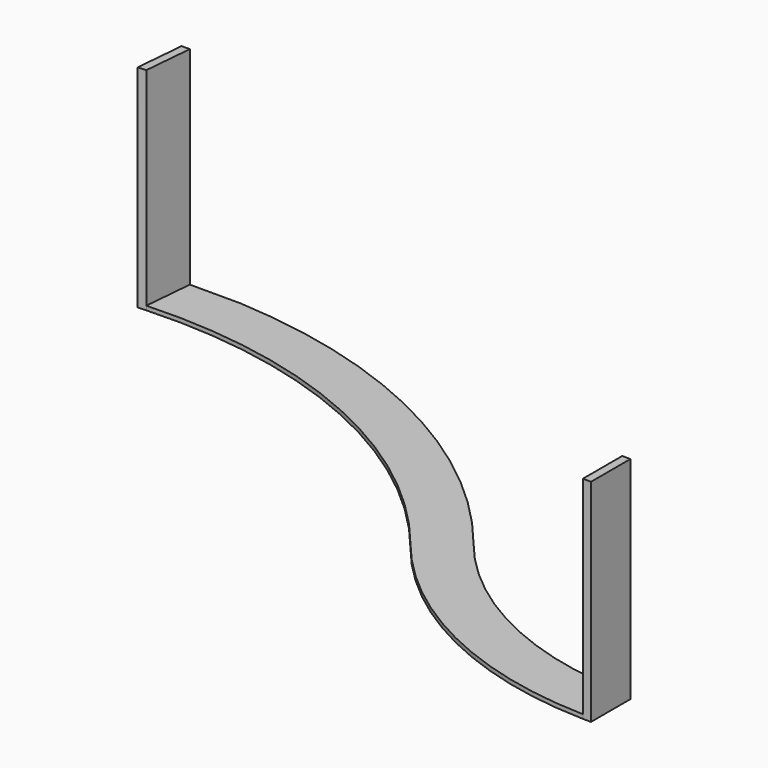
from build123d import *

# Parameters (mm, degrees)
F1_DEPTH = 25.4
F2_DEPTH = 1308.1
F3_DEPTH = 25.4
F4_DEPTH = 1308.1


with BuildPart() as f1:
    # F0 (on Top) → F1 (new body)
    with BuildSketch(Plane.XY):
        with BuildLine():
            Line((-1948.5691277788, 99.7355101007), (-2263.234400171, 99.7355101007))
            Line((-2263.234400171, 99.7355101007), (-2289.862411819, -203.7745007557))
            ThreePointArc((-2289.862411819, -203.7745007557), (-874.5398284023, -470.4550472357), (263.8832180742, -1352.6395496224))
            ThreePointArc((263.8832180742, -1352.6395496224), (346.7538874408, -1450.5053929427), (434.8963853674, -1543.651360055))
            Line((434.8963853674, -1543.651360055), (650.422532273, -1328.1252131493))
            ThreePointArc((650.422532273, -1328.1252131493), (573.8397062056, -1247.1951105763), (501.8373213462, -1162.1641319538))
            ThreePointArc((501.8373213462, -1162.1641319538), (-588.8138343544, -269.9358016898), (-1948.5691277788, 99.7355101007))
        make_face()
    extrude(amount=F1_DEPTH)

    # F0 (on Top) → F2 (join)
    with BuildSketch(Plane.XY):
        with BuildLine():
            Line((-2263.234400171, 99.7355101007), (-2314.2295336755, 99.7355101007))
            Line((-2314.2295336755, 99.7355101007), (-2341.1214825581, -206.7828963515))
            ThreePointArc((-2341.1214825581, -206.7828963515), (-2315.4982300933, -205.1716461899), (-2289.862411819, -203.7745007557))
            Line((-2289.862411819, -203.7745007557), (-2263.234400171, 99.7355101007))
        make_face()
    extrude(amount=F2_DEPTH)

    # F0 (on Top) → F3 (join)
    with BuildSketch(Plane.XY):
        with BuildLine():
            ThreePointArc((2027.483255523, -1918.925395054), (1282.1233486229, -1755.9858840328), (650.422532273, -1328.1252131493))
            Line((650.422532273, -1328.1252131493), (434.8963853674, -1543.651360055))
            ThreePointArc((434.8963853674, -1543.651360055), (1165.4738720531, -2037.6039199968), (2027.483255523, -2223.8092323134))
            Line((2027.483255523, -2223.8092323134), (2027.483255523, -1918.925395054))
        make_face()
    extrude(amount=F3_DEPTH)

    # F0 (on Top) → F4 (join)
    with BuildSketch(Plane.XY):
        with BuildLine():
            ThreePointArc((2052.883255523, -1919.4047351522), (2040.182501702, -1919.2050097162), (2027.483255523, -1918.925395054))
            Line((2027.483255523, -1918.925395054), (2027.483255523, -2223.8092323134))
            ThreePointArc((2027.483255523, -2223.8092323134), (2052.8817382899, -2224.225671357), (2078.283255523, -2224.3644898993))
            Line((2078.283255523, -2224.3644898993), (2078.283255523, -1919.5644898993))
            ThreePointArc((2078.283255523, -1919.5644898993), (2065.5830043289, -1919.5245508176), (2052.883255523, -1919.4047351522))
        make_face()
    extrude(amount=F4_DEPTH)


solid = f1.part
